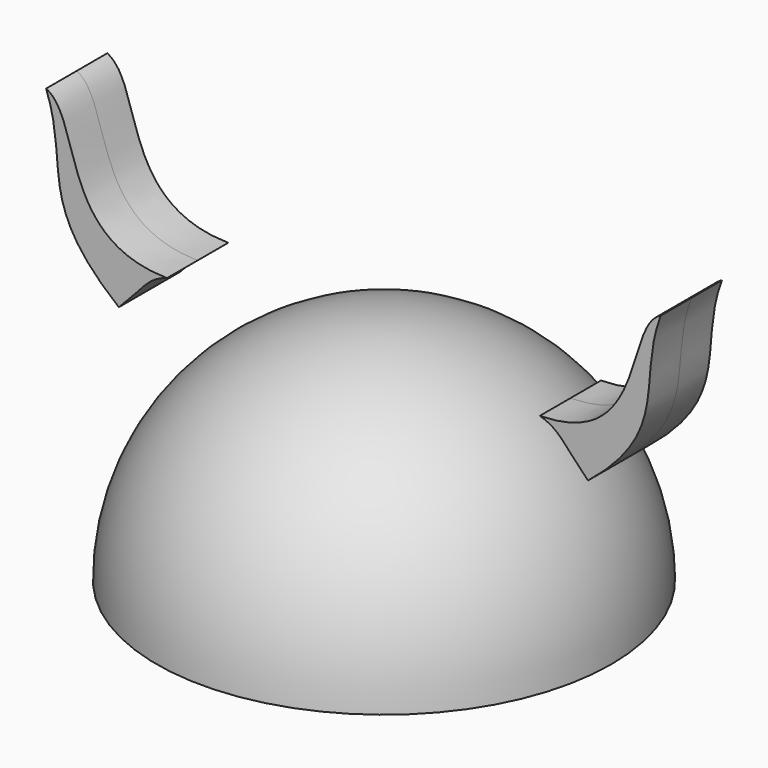
from build123d import *

# Parameters (mm, degrees)
F3_DEPTH = 6.35


# Not quite as in the source:
# - the program builds the solid bodies; features that only make, move or delete a surface that nothing else refers to are left out


with BuildPart() as f1:
    # F0 (on Front) → F1 (revolve)
    with BuildSketch(Plane.XZ):
        with BuildLine():
            Line((0, 33.5709042847), (0, 37.7536378801))
            ThreePointArc((0, 37.7536378801), (-26.6958533595, 26.6958533595), (-37.7536378801, 0))
            Line((-37.7536378801, 0), (-33.5709042847, 0))
            ThreePointArc((-33.5709042847, 0), (-23.7382140703, 23.7382140703), (0, 33.5709042847))
        make_face()
    revolve(axis=Axis((0, 0, 18.87681894), (0, 0, -1)))


with BuildPart() as f3:
    # F2 (on Front) → F3 (new body, symmetric)
    with BuildSketch(Plane.XZ):
        with BuildLine():
            add(Edge.make_bspline(
                [(30.9544112533, 36.6997048259), (48.9418655634, 36.9769893587), (44.9549630284, 54.9721755087), (51.0374158621, 57.8818283975)],
                knots=[0, 0, 0, 0, 29.1892006249, 29.1892006249, 29.1892006249, 29.1892006249], degree=3))
            add(Edge.make_bspline(
                [(30.9544112533, 36.6997048259), (34.3832373619, 35.7200428843), (35.0363478065, 33.5974358022), (38.9550067484, 29.842056334)],
                knots=[0, 0, 0, 0, 10.5374034332, 10.5374034332, 10.5374034332, 10.5374034332], degree=3))
            add(Edge.make_bspline(
                [(38.9550067484, 29.842056334), (52.9238283634, 41.034411639), (47.0328231653, 47.3239459097), (51.0374158621, 57.8818283975)],
                knots=[0, 0, 0, 0, 30.5321703677, 30.5321703677, 30.5321703677, 30.5321703677], degree=3))
        make_face()
    extrude(amount=F3_DEPTH, both=True)


with BuildPart() as f3b:
    # F2 (on Front) → F3, piece 2 (new body, symmetric)
    with BuildSketch(Plane.XZ):
        with BuildLine():
            add(Edge.make_bspline(
                [(-38.9550067484, 29.842056334), (-52.9238283634, 41.034411639), (-47.0328231653, 47.3239459097), (-51.0374158621, 57.8818283975)],
                knots=[0, 0, 0, 0, 30.5321703677, 30.5321703677, 30.5321703677, 30.5321703677], degree=3))
            add(Edge.make_bspline(
                [(-30.9544112533, 36.6997048259), (-34.3832373619, 35.7200428843), (-35.0363478065, 33.5974358022), (-38.9550067484, 29.842056334)],
                knots=[0, 0, 0, 0, 10.5374034332, 10.5374034332, 10.5374034332, 10.5374034332], degree=3))
            add(Edge.make_bspline(
                [(-30.9544112533, 36.6997048259), (-48.9418655634, 36.9769893587), (-44.9549630284, 54.9721755087), (-51.0374158621, 57.8818283975)],
                knots=[0, 0, 0, 0, 29.1892006249, 29.1892006249, 29.1892006249, 29.1892006249], degree=3))
        make_face()
    extrude(amount=F3_DEPTH, both=True)


solid = Compound([f1.part, f3.part, f3b.part])
